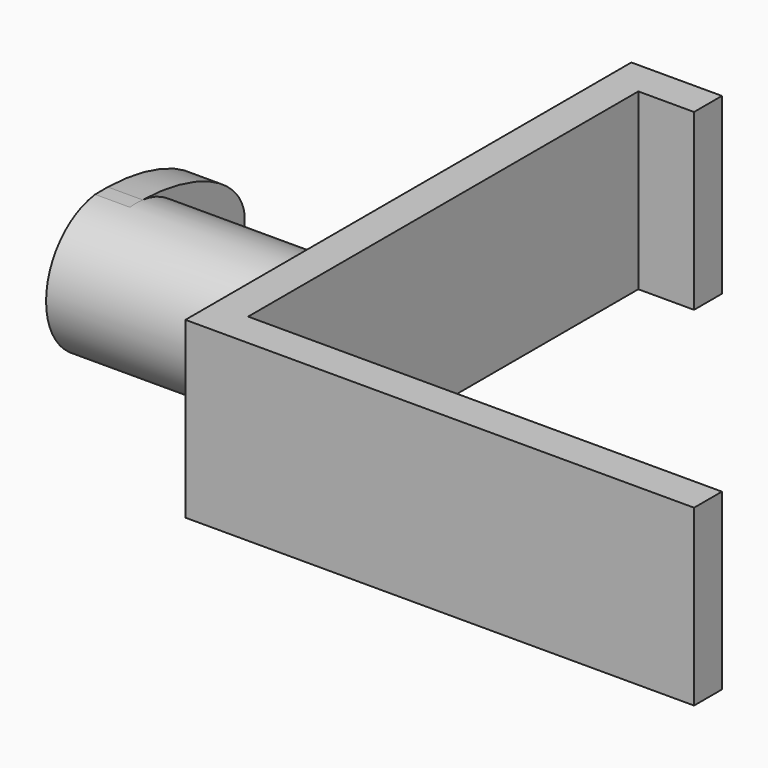
from build123d import *

# Parameters (mm, degrees)
F1_DEPTH = 12.5
F3_DEPTH = 25
F5_DEPTH = 5


with BuildPart() as f1:
    # F0 (on Top) → F1 (new body, symmetric)
    with BuildSketch(Plane.XY):
        Polygon((3.3505584225, 19.8199842125), (-9.6494415775, 19.8199842125), (-9.6494415775, -60.1800157875), (63.3505584225, -60.1800157875), (63.3505584225, -55.1800157875), (-4.6494415775, -55.1800157875), (-4.6494415775, 14.8199842125), (3.3505584225, 14.8199842125), align=None)
    extrude(amount=F1_DEPTH, both=True)

    # F2 (on face) → F3 (join)
    with BuildSketch(Plane(origin=(-9.6494415775, 0, 0), x_dir=(0, -1, 0), z_dir=(-1, 0, 0))):
        with BuildLine():
            ThreePointArc((47.6800157875, 0), (46.3402698253, 5), (42.6800157875, 8.6602540378))
            ThreePointArc((42.6800157875, 8.6602540378), (37.6800157875, 0), (42.6800157875, -8.6602540378))
            ThreePointArc((42.6800157875, -8.6602540378), (46.3402698253, -5), (47.6800157875, 0))
        make_face()
        with BuildLine():
            ThreePointArc((42.6800157875, -8.6602540378), (37.6800157875, 0), (42.6800157875, 8.6602540378))
            ThreePointArc((42.6800157875, 8.6602540378), (27.6800157875, 0), (42.6800157875, -8.6602540378))
        make_face()
    extrude(amount=F3_DEPTH)

    # F4 (on face) → F5 (join)
    with BuildSketch(Plane(origin=(-34.6494415775, 0, 0), x_dir=(0, -1, 0), z_dir=(-1, 0, 0))):
        with BuildLine():
            add(Edge.make_bspline(
                [(36.6172563189, 9.9433667493), (18.2870905846, 9.5103947751), (18.2870905846, 0)],
                knots=[4.7579309047, 4.7579309047, 4.7579309047, 6.2831853072, 6.2831853072, 6.2831853072], degree=2, weights=[1, 0.7230235761, 1]))
            add(Edge.make_bspline(
                [(18.2870905846, 0), (18.2870905846, -9.5103947751), (36.6172563189, -9.9433667493)],
                knots=[0, 0, 0, 1.5252544025, 1.5252544025, 1.5252544025], degree=2, weights=[1, 0.7230235761, 1]))
            ThreePointArc((36.6172563189, -9.9433667493), (27.6800157875, 0), (36.6172563189, 9.9433667493))
        make_face()
        with BuildLine():
            ThreePointArc((36.6172563189, 9.9433667493), (27.6800157875, 0), (36.6172563189, -9.9433667493))
            add(Edge.make_bspline(
                [(36.6172563189, -9.9433667493), (37.750134496, -9.9701261637), (38.8812156146, -9.927593816)],
                knots=[1.5252544025, 1.5252544025, 1.5252544025, 1.6432205296, 1.6432205296, 1.6432205296], degree=2, weights=[1, 0.9982610034, 1]))
            ThreePointArc((38.8812156146, -9.927593816), (45.1637313844, -6.6327973634), (47.6800157875, 0))
            ThreePointArc((47.6800157875, 0), (45.1637313844, 6.6327973634), (38.8812156146, 9.927593816))
            add(Edge.make_bspline(
                [(38.8812156146, 9.927593816), (37.750134496, 9.9701261637), (36.6172563189, 9.9433667493)],
                knots=[4.6399647776, 4.6399647776, 4.6399647776, 4.7579309047, 4.7579309047, 4.7579309047], degree=2, weights=[1, 0.9982610034, 1]))
        make_face()
    extrude(amount=F5_DEPTH)


solid = f1.part
